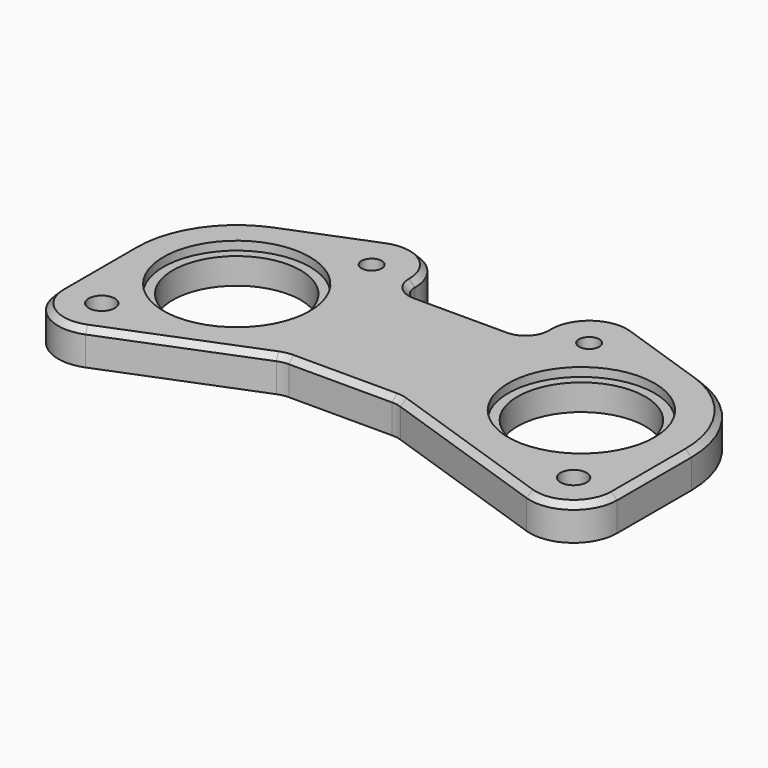
from build123d import *

# Parameters (mm, degrees)
F0_R     = 4.5
F0_R_2   = 22
F0_R_3   = 3.5
F1_DEPTH = 12
F2_R     = 25.2
F3_DEPTH = 3
F4_SIZE  = 2


# Not quite as in the source:
# - ends of sketch curves that miss each other by under 0.0002 mm in the source are joined


with BuildPart() as f1:
    # F0 (on Top) → F1 (new body)
    with BuildSketch(Plane.XY):
        with BuildLine():
            Line((-96.25, -7.835472), (-96.25, -39.300472))
            ThreePointArc((-96.25, -39.300472), (-89.6603385796, -51.720866719), (-75.6811726698, -53.2284353172))
            Line((-75.6811726698, -53.2284353172), (-25.901923657, -33.3251628629))
            ThreePointArc((-25.901923657, -33.3251628629), (-24.0797305928, -32.7907701516), (-22.189372, -32.610472))
            Line((-22.189372, -32.610472), (13.41096, -32.610472))
            ThreePointArc((13.41096, -32.610472), (15.0445629213, -32.7448072228), (16.6342757601, -33.1442037009))
            Line((16.6342757601, -33.1442037009), (76.4150264593, -53.4998741564))
            ThreePointArc((76.4150264593, -53.4998741564), (89.9814201421, -51.4972872524), (96.25, -39.300472))
            Line((96.25, -39.300472), (96.25, -7.385472))
            ThreePointArc((96.25, -7.385472), (89.1771507076, 14.6451910108), (70.602136617, 28.4417181588))
            Line((70.602136617, 28.4417181588), (40.3905414757, 38.7289301785))
            ThreePointArc((40.3905414757, 38.7289301785), (26.82414783, 36.7263432324), (20.555568, 24.529528))
            Line((20.555568, 24.529528), (20.555568, 23.389528))
            ThreePointArc((20.555568, 23.389528), (18.7982086871, 19.1468873129), (14.555568, 17.389528))
            Line((14.555568, 17.389528), (-17.637618, 17.389528))
            ThreePointArc((-17.637618, 17.389528), (-21.8802586871, 19.1468873129), (-23.637618, 23.389528))
            Line((-23.637618, 23.389528), (-23.637618, 23.629528))
            ThreePointArc((-23.637618, 23.629528), (-30.2272793638, 36.0499226807), (-44.2064452032, 37.557491368))
            Line((-44.2064452032, 37.557491368), (-73.4226694122, 25.875948235))
            ThreePointArc((-73.4226694122, 25.875948235), (-90.0062904382, 12.5210187268), (-96.25, -7.835472))
        make_face()
        with Locations((-81.25, -39.300472)):
            Circle(F0_R, mode=Mode.SUBTRACT)
        with Locations((-59.943809, -7.835472)):
            Circle(F0_R_2, mode=Mode.SUBTRACT)
        with Locations((81.25, -39.300472)):
            Circle(F0_R, mode=Mode.SUBTRACT)
        with Locations((-38.637618, 23.629528)):
            Circle(F0_R_3, mode=Mode.SUBTRACT)
        with Locations((58.402784, -7.385472)):
            Circle(F0_R_2, mode=Mode.SUBTRACT)
        with Locations((35.555568, 24.529528)):
            Circle(F0_R_3, mode=Mode.SUBTRACT)
    extrude(amount=F1_DEPTH)

    # F2 (on face) → F3 (cut)
    with BuildSketch(Plane.XY.offset(12)):
        with Locations((-59.943809, -7.835472)):
            Circle(F2_R)
        with Locations((58.402784, -7.385472)):
            Circle(F2_R)
    extrude(amount=-F3_DEPTH, mode=Mode.SUBTRACT)

    # F4
    f4_edges = [f1.edges().sort_by_distance(p)[0] for p in [
        (-58.814557, 31.71672, 12),
    ]]
    chamfer(f4_edges, length=F4_SIZE)


solid = f1.part
